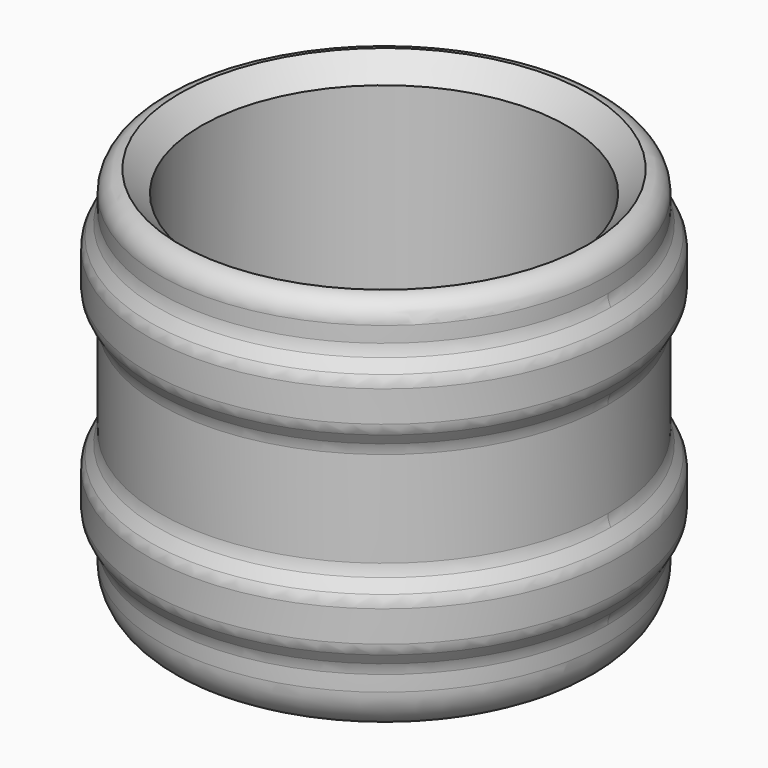
from build123d import *

# Parameters (mm, degrees)
F0_R     = 16.51
F1_DEPTH = 9.525
F2_R     = 16.51
F2_R_2   = 13.49375
F3_DEPTH = 19.05
F4_SIZE  = 1.5875
F6_R     = 3.175
F9_R     = 1.5875


# Not quite as in the source:
# - a fillet or chamfer that OpenCascade refuses, or shapes differently, is made with other operations: its cross-section is extruded or revolved along the edge and cut away or added


with BuildPart() as f1:
    # F0 (on Top) → F1 (new body)
    with BuildSketch(Plane.XY):
        Circle(F0_R)
        with BuildLine():
            ThreePointArc((3.4919226796, 1.524), (0, -3.81), (-3.4919226796, 1.524))
            Line((-3.4919226796, 1.524), (3.4919226796, 1.524))
        make_face(mode=Mode.SUBTRACT)
    extrude(amount=F1_DEPTH)

    # F2 (on face) → F3 (join)
    with BuildSketch(Plane.XY.offset(9.525)):
        Circle(F2_R)
        Circle(F2_R_2, mode=Mode.SUBTRACT)
    extrude(amount=F3_DEPTH)

    # F4
    f4_edges = [f1.edges().sort_by_distance(p)[0] for p in [
        (-13.49375, 0, 28.575),
    ]]
    chamfer(f4_edges, length=F4_SIZE)

    # F5: fillet of radius 1.5875 on 1 edges, made by hand

    # F5_s1 → F5_t2 (revolve, cut)
    with BuildSketch(Plane.XZ):
        with BuildLine():
            ThreePointArc((15.08125, 28.575), (16.0998215098, 28.0603848179), (16.51, 26.9954574436))
            Line((16.51, 26.9954574436), (16.51, 28.575))
            Line((16.51, 28.575), (15.08125, 28.575))
        make_face()
    revolve(axis=Axis((0, 0, 28.575), (0, 0, 1)), mode=Mode.SUBTRACT)

    # F6
    f6_edges = [f1.edges().sort_by_distance(p)[0] for p in [
        (-16.51, 0, 0),
    ]]
    fillet(f6_edges, radius=F6_R)

    # F7 (on Right) → F8 (revolve)
    with BuildSketch(Plane.YZ):
        Polygon((17.4625, 23.8125), (16.51, 25.4), (16.51, 19.05), (17.4625, 20.6375), align=None)
        Polygon((17.4625, 9.525), (16.51, 11.1125), (16.51, 4.7625), (17.4625, 6.35), align=None)
    revolve(axis=Axis((0, 0, 15.1199988206), (0, 0, -1)))

    # F9
    f9_edges = [f1.edges().sort_by_distance(p)[0] for p in [
        (0, -17.4625, 23.8125),
        (16.51, 0, 26.197729),
        (0, -17.4625, 20.6375),
        (-11.674333, -11.674333, 19.05),
        (16.51, 0, 15.08125),
        (0, -17.4625, 9.525),
        (0, -17.4625, 6.35),
        (-11.674333, -11.674333, 4.7625),
        (11.674333, 11.674333, 25.4),
        (-11.674333, -11.674333, 25.4),
        (11.674333, 11.674333, 19.05),
        (11.674333, 11.674333, 11.1125),
        (-11.674333, -11.674333, 11.1125),
        (11.674333, 11.674333, 4.7625),
    ]]
    fillet(f9_edges, radius=F9_R)


solid = f1.part
